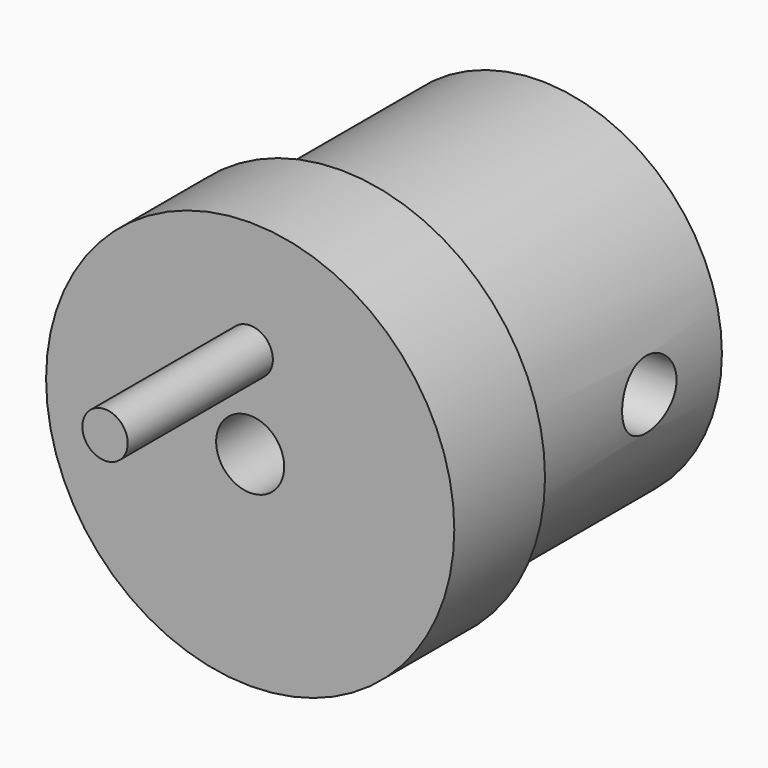
from build123d import *

# Parameters (mm, degrees)
F0_R          = 9
F0_R_2        = 8
F1_DEPTH      = 5
F2_DEPTH      = 11
F3_R          = 2.5
F4_DEPTH      = 0.5
F5_R          = 1.5
F6_DEPTH      = 25
F5_R_2        = 1
F7_DEPTH      = 8
F8_R          = 1.5
F9_DEPTH      = 9.001
F9_DEPTH_BACK = 9.001


with BuildPart() as f1:
    # F0 (on Front) → F1 (new body)
    with BuildSketch(Plane.XZ):
        Circle(F0_R)
        Circle(F0_R_2, mode=Mode.SUBTRACT)
        Circle(F0_R_2)
    extrude(amount=F1_DEPTH)

    # F0 (on Front) → F2 (join)
    with BuildSketch(Plane.XZ):
        Circle(F0_R_2)
    extrude(amount=-F2_DEPTH)

    # F3 (on face) → F4 (join)
    with BuildSketch(Plane(origin=(0, 11, 0), x_dir=(-1, 0, 0), z_dir=(0, 1, 0))):
        Circle(F3_R)
    extrude(amount=F4_DEPTH)

    # F5 (on face) → F6 (cut)
    with BuildSketch(Plane.XZ.offset(5)):
        Circle(F5_R)
    extrude(amount=-F6_DEPTH, mode=Mode.SUBTRACT)

    # F5 (on face) → F7 (join)
    with BuildSketch(Plane.XZ.offset(5)):
        with Locations((0, 4)):
            Circle(F5_R_2)
    extrude(amount=F7_DEPTH)

    # F8 (on Right) → F9 (cut, two sides)
    with BuildSketch(Plane.YZ) as f9_sk:
        with Locations((7, 0)):
            Circle(F8_R)
    extrude(amount=-F9_DEPTH, mode=Mode.SUBTRACT)
    extrude(f9_sk.sketch, amount=F9_DEPTH_BACK, mode=Mode.SUBTRACT)


solid = f1.part
